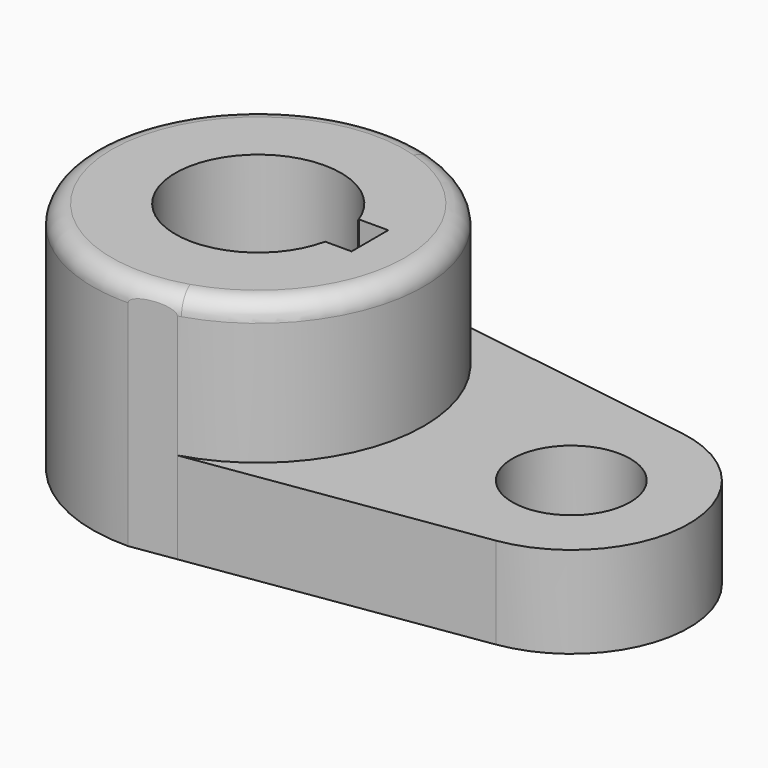
from build123d import *

# Parameters (mm, degrees)
F1_DEPTH    = 40.2336
F0_R        = 10.16
F2_DEPTH    = 15.7734
F3_T2_ANGLE = 214.9193133158
F3_T4_ANGLE = 180.6316694895


# Not quite as in the source:
# - a fillet or chamfer that OpenCascade refuses, or shapes differently, is made with other operations: its cross-section is extruded or revolved along the edge and cut away or added


with BuildPart() as f1:
    # F0 (on Top) → F1 (new body)
    with BuildSketch(Plane.XY):
        with BuildLine():
            Line((-37.0835625183, 27.4328460411), (-44.6425986707, 28.5716266437))
            ThreePointArc((-44.6425986707, 28.5716266437), (-73.6566612351, 0), (-44.6425986707, -28.5716266437))
            Line((-44.6425986707, -28.5716266437), (-37.0835625183, -27.4328460411))
            ThreePointArc((-37.0835625183, -27.4328460411), (-22.2225679041, -17.1462088254), (-16.5066612351, 0))
            ThreePointArc((-16.5066612351, 0), (-22.2225679041, 17.1462088254), (-37.0835625183, 27.4328460411))
        make_face()
        with BuildLine():
            ThreePointArc((-31.1201480581, -3.0346014662), (-59.3439011555, -0.8492165229), (-31.5788975811, 4.6699068463))
            Line((-31.5788975811, 4.6699068463), (-31.5788975811, 4.8789530993))
            Line((-31.5788975811, 4.8789530993), (-26.5667859032, 4.8789530993))
            Line((-26.5667859032, 4.8789530993), (-26.5667859032, 4.6699068463))
            Line((-26.5667859032, 4.6699068463), (-26.5667859032, 0.7309924323))
            Line((-26.5667859032, 0.7309924323), (-26.5667859032, -3.0346014662))
            Line((-26.5667859032, -3.0346014662), (-31.1201480581, -3.0346014662))
        make_face(mode=Mode.SUBTRACT)
    extrude(amount=F1_DEPTH)

    # F0 (on Top) → F2 (join)
    with BuildSketch(Plane.XY):
        with BuildLine():
            Line((11.9140942867, 20.051272516), (-37.0835625183, 27.4328460411))
            ThreePointArc((-37.0835625183, 27.4328460411), (-22.2225679041, 17.1462088254), (-16.5066612351, 0))
            ThreePointArc((-16.5066612351, 0), (-22.2225679041, -17.1462088254), (-37.0835625183, -27.4328460411))
            Line((-37.0835625183, -27.4328460411), (11.9140942867, -20.051272516))
            ThreePointArc((11.9140942867, -20.051272516), (29.1708754356, 0), (11.9140942867, 20.051272516))
        make_face()
        with Locations((8.8933387649, 0)):
            Circle(F0_R, mode=Mode.SUBTRACT)
    extrude(amount=F2_DEPTH)

    # F3: fillet of radius 3.302 on 2 edges, made by hand

    # F3_s1 → F3_t2 (revolve, cut)
    with BuildSketch(Plane(origin=(-41.0233868693, 12.9028740724, 0), x_dir=(0, 0, 1), z_dir=(0.9539284485, -0.3000341899, 0))):
        with BuildLine():
            ThreePointArc((36.9316, -15.048960293), (39.2664665915, -14.0818268845), (40.2336, -11.746960293))
            Line((40.2336, -11.746960293), (40.2336, -15.048960293))
            Line((40.2336, -15.048960293), (36.9316, -15.048960293))
        make_face()
    revolve(axis=Axis((-45.0816612351, 0, 40.2336), (0, 0, 1)), revolution_arc=F3_T2_ANGLE, mode=Mode.SUBTRACT)

    # F3_s3 → F3_t4 (revolve, cut)
    with BuildSketch(Plane(origin=(-45.0802913944, -0.2485011402, 0), x_dir=(0, 0, 1), z_dir=(-0.999984807, -0.0055123283, 0))):
        with BuildLine():
            ThreePointArc((40.2336, 25.5215049158), (39.2664665915, 27.8563715073), (36.9316, 28.8235049158))
            Line((36.9316, 28.8235049158), (40.2336, 28.8235049158))
            Line((40.2336, 28.8235049158), (40.2336, 25.5215049158))
        make_face()
    revolve(axis=Axis((-45.0816612351, 0, 40.2336), (0, 0, -1)), revolution_arc=F3_T4_ANGLE, mode=Mode.SUBTRACT)


solid = f1.part
